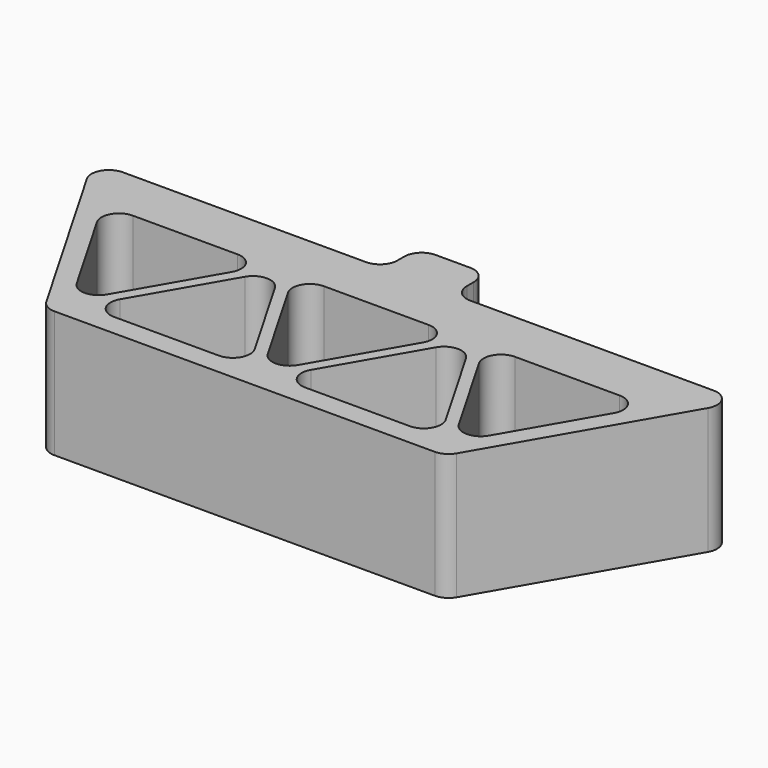
from build123d import *

# Parameters (mm, degrees)
F0_W           = 20.32
F0_H           = 12.7
F1_DEPTH       = 37.084
F5_D           = 9.525
F5_DEPTH       = 6.35
F5_TIP         = 2.8615986981
F5_ON_F3_D     = 9.525
F5_ON_F3_DEPTH = 6.35
F5_ON_F3_TIP   = 2.8615986981
F5_ON_F4_D     = 9.525
F5_ON_F4_DEPTH = 6.35
F5_ON_F4_TIP   = 2.8615986981
F7_DEPTH       = 37.085
F8_R           = 5.08


# Not quite as in the source:
# - a length typed as a fraction of an inch, garbled in the dataset ("3 / 203.2 mm" for 3/8 in), is restored


with BuildPart() as f1:
    # F0 (on Top) → F1 (new body)
    with BuildSketch(Plane.XY):
        with Locations((58.5882579065, 69.85)):
            Rectangle(F0_W, F0_H)
        Polygon((48.4282579065, 63.5), (-36.6617420935, 63.5), (0, 0), (117.1765158129, 0), (153.8382579065, 63.5), (68.7482579065, 63.5), align=None)
    extrude(amount=F1_DEPTH)

    # F5
    with Locations(Plane(origin=(0, 63.5, 0), x_dir=(-1, 0, 0), z_dir=(0, 1, 0))):
        with Locations((-136.8202579065, 18.542), (-119.8022579065, 18.542), (-102.7842579065, 18.542), (-85.7662579065, 18.542)):
            Hole(F5_D / 2, depth=F5_DEPTH)
            with Locations((0, 0, -(F5_DEPTH + F5_TIP / 2))):  # 118° drill point
                Cone(0, F5_D / 2, F5_TIP, mode=Mode.SUBTRACT)

    # F5 on F3
    with Locations(Plane(origin=(0, 63.5, 0), x_dir=(-1, 0, 0), z_dir=(0, 1, 0))):
        with Locations((-31.4102579065, 18.542), (-14.3922579065, 18.542), (2.6257420935, 18.542), (19.6437420935, 18.542)):
            Hole(F5_ON_F3_D / 2, depth=F5_ON_F3_DEPTH)
            with Locations((0, 0, -(F5_ON_F3_DEPTH + F5_ON_F3_TIP / 2))):  # 118° drill point
                Cone(0, F5_ON_F3_D / 2, F5_ON_F3_TIP, mode=Mode.SUBTRACT)

    # F5 on F4
    with Locations(Plane(origin=(0, 76.2, 0), x_dir=(-1, 0, 0), z_dir=(0, 1, 0))):
        with Locations((-58.5882579065, 18.542)):
            Hole(F5_ON_F4_D / 2, depth=F5_ON_F4_DEPTH)
            with Locations((0, 0, -(F5_ON_F4_DEPTH + F5_ON_F4_TIP / 2))):  # 118° drill point
                Cone(0, F5_ON_F4_D / 2, F5_ON_F4_TIP, mode=Mode.SUBTRACT)

    # F6 (on face) → F7 (cut, through all)
    with BuildSketch(Plane.XY.offset(37.084)):
        Polygon((26.8260418486, 48.1655448196), (-21.4583902673, 48.1655448196), (2.6838257906, 6.35), align=None)
        Polygon((54.7782579065, 6.35), (30.6360418486, 48.1655448196), (6.4938257906, 6.35), align=None)
        Polygon((82.7304739644, 48.1655448196), (34.4460418486, 48.1655448196), (58.5882579065, 6.35), align=None)
        Polygon((110.6826900223, 6.35), (86.5404739644, 48.1655448196), (62.3982579065, 6.35), align=None)
        Polygon((138.6349060802, 48.1655448196), (90.3504739644, 48.1655448196), (114.4926900223, 6.35), align=None)
    extrude(amount=-F7_DEPTH, mode=Mode.SUBTRACT)

    # F8
    f8_edges = [f1.edges().sort_by_distance(p)[0] for p in [
        (48.428258, 63.5, 18.542),
        (68.748258, 63.5, 18.542),
        (48.428258, 76.2, 18.542),
        (68.748258, 76.2, 18.542),
        (153.838258, 63.5, 18.542),
        (-36.661742, 63.5, 18.542),
        (-21.45839, 48.165545, 18.542),
        (0, 0, 18.542),
        (26.826042, 48.165545, 18.542),
        (82.730474, 48.165545, 18.542),
        (138.634906, 48.165545, 18.542),
        (110.68269, 6.35, 18.542),
        (114.49269, 6.35, 18.542),
        (2.683826, 6.35, 18.542),
        (117.176516, 0, 18.542),
        (90.350474, 48.165545, 18.542),
        (34.446042, 48.165545, 18.542),
        (30.636042, 48.165545, 18.542),
        (86.540474, 48.165545, 18.542),
        (62.398258, 6.35, 18.542),
        (6.493826, 6.35, 18.542),
        (58.588258, 6.35, 18.542),
        (54.778258, 6.35, 18.542),
    ]]
    fillet(f8_edges, radius=F8_R)


solid = f1.part
